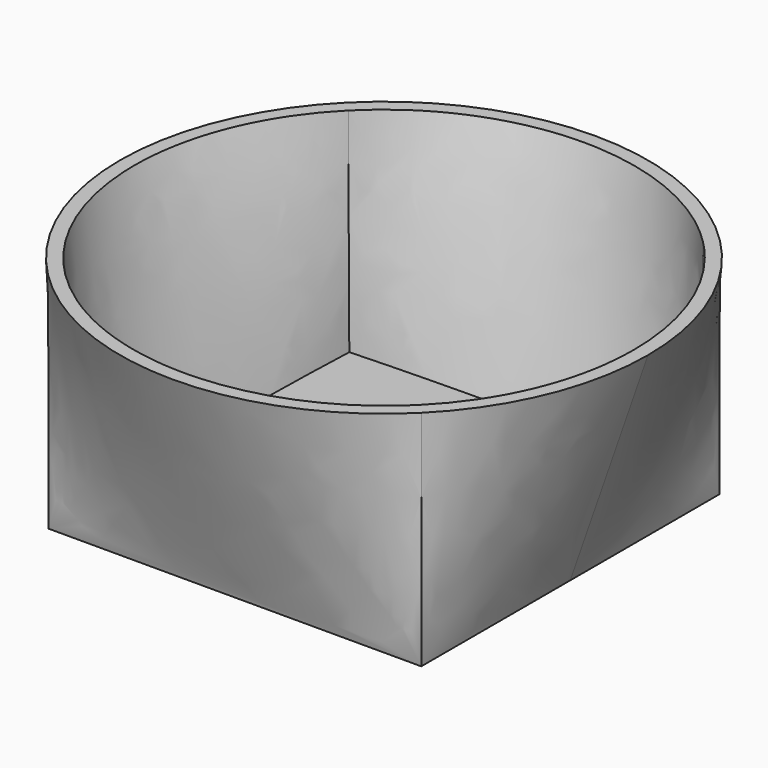
from build123d import *

# Parameters (mm, degrees)
F0_W = 50
F0_H = 50
F2_R = 35.4285378843
F4_T = 1.8


# Not quite as in the source:
# - a shell that OpenCascade refuses in one call is made with other operations: the cavity is built on its own and cut out


with BuildPart() as f3:
    # F0 (on Top) → F3 section 0
    with BuildSketch(Plane.XY):
        Rectangle(F0_W, F0_H)
    # F2 (on offset) → F3 section 1
    with BuildSketch(Plane.XY.offset(30)):
        Circle(F2_R)
    loft()

    # F4: shell of thickness 1.8, made by hand


with BuildPart() as f4_core1:
    # F4_t2: copy of F3
    add(f3.part)

    # the walls: a layer under each face that stays
    f4_faces = [f4_core1.faces().sort_by_distance(p)[0] for p in [
        (0, 30.2142689408, 15),
        (-30.2142689408, 0, 15),
        (0, -30.2142689408, 15),
        (28.8658505055, -13.0289572392, 15),
        (28.8658505055, 13.0289572392, 15),
        (0, 0, 0),
    ]]
    thicken(f4_faces, amount=-F4_T, mode=Mode.SUBTRACT)


with BuildPart() as f3_1:
    add(f3.part)

    # what is left inside the walls is the cavity
    f4_cavity = [f4_core1.part.solids().sort_by_distance(p)[0] for p in [
        (0, -11.174295, 29.982),
    ]]
    add(f4_cavity, mode=Mode.SUBTRACT)


solid = f3_1.part
